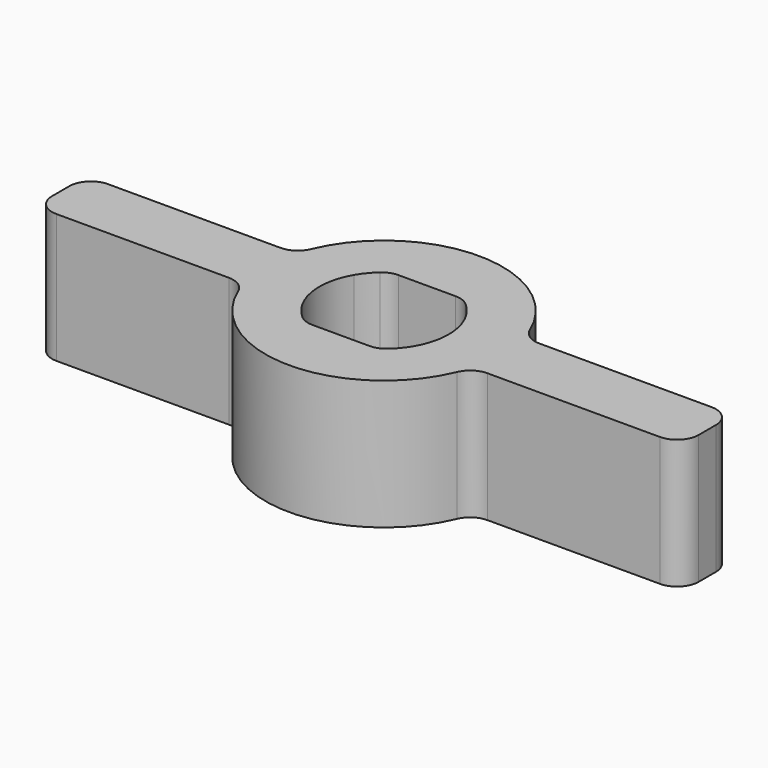
from build123d import *

# Parameters (mm, degrees)
F1_DEPTH = 6
F2_R     = 1
F3_R     = 1


with BuildPart() as f1:
    # F0 (on Top) → F1 (new body)
    with BuildSketch(Plane.XY):
        with BuildLine():
            ThreePointArc((-5.2915026221, -1.5), (0, -5.5), (5.2915026221, -1.5))
            Line((5.2915026221, -1.5), (2.5980762114, -1.5))
            ThreePointArc((2.5980762114, -1.5), (2.1861406616, -2.0544558909), (1.6583123952, -2.5))
            ThreePointArc((1.6583123952, -2.5), (0, -3), (-1.6583123952, -2.5))
            ThreePointArc((-1.6583123952, -2.5), (-2.1861406616, -2.0544558909), (-2.5980762114, -1.5))
            Line((-2.5980762114, -1.5), (-5.2915026221, -1.5))
        make_face()
        with BuildLine():
            ThreePointArc((-5.2915026221, -1.5), (-5.5, 0), (-5.2915026221, 1.5))
            Line((-5.2915026221, 1.5), (-15, 1.5))
            Line((-15, 1.5), (-15, -1.5))
            Line((-15, -1.5), (-5.2915026221, -1.5))
        make_face()
        with BuildLine():
            Line((-2.5980762114, 1.5), (-5.2915026221, 1.5))
            ThreePointArc((-5.2915026221, 1.5), (-5.5, 0), (-5.2915026221, -1.5))
            Line((-5.2915026221, -1.5), (-2.5980762114, -1.5))
            ThreePointArc((-2.5980762114, -1.5), (-3, 0), (-2.5980762114, 1.5))
        make_face()
        with BuildLine():
            ThreePointArc((5.2915026221, 1.5), (5.4476262914, 0.7572105316), (5.5, 0))
            ThreePointArc((5.5, 0), (5.4476262914, -0.7572105316), (5.2915026221, -1.5))
            Line((5.2915026221, -1.5), (15, -1.5))
            Line((15, -1.5), (15, 1.5))
            Line((15, 1.5), (5.2915026221, 1.5))
        make_face()
        with BuildLine():
            ThreePointArc((5.2915026221, -1.5), (5.4476262914, -0.7572105316), (5.5, 0))
            ThreePointArc((5.5, 0), (5.4476262914, 0.7572105316), (5.2915026221, 1.5))
            Line((5.2915026221, 1.5), (2.5980762114, 1.5))
            ThreePointArc((2.5980762114, 1.5), (2.8977774789, 0.7764571353), (3, 0))
            ThreePointArc((3, 0), (2.8977774789, -0.7764571353), (2.5980762114, -1.5))
            Line((2.5980762114, -1.5), (5.2915026221, -1.5))
        make_face()
        with BuildLine():
            Line((2.5980762114, 1.5), (5.2915026221, 1.5))
            ThreePointArc((5.2915026221, 1.5), (0, 5.5), (-5.2915026221, 1.5))
            Line((-5.2915026221, 1.5), (-2.5980762114, 1.5))
            ThreePointArc((-2.5980762114, 1.5), (-2.1861406616, 2.0544558909), (-1.6583123952, 2.5))
            ThreePointArc((-1.6583123952, 2.5), (0, 3), (1.6583123952, 2.5))
            ThreePointArc((1.6583123952, 2.5), (2.1861406616, 2.0544558909), (2.5980762114, 1.5))
        make_face()
        with BuildLine():
            Line((-1.6583123952, 2.5), (1.6583123952, 2.5))
            ThreePointArc((1.6583123952, 2.5), (0, 3), (-1.6583123952, 2.5))
        make_face()
        with BuildLine():
            ThreePointArc((-1.6583123952, -2.5), (0, -3), (1.6583123952, -2.5))
            Line((1.6583123952, -2.5), (-1.6583123952, -2.5))
        make_face()
    extrude(amount=F1_DEPTH)

    # F2
    f2_edges = [f1.edges().sort_by_distance(p)[0] for p in [
        (15, -1.5, 3),
        (-15, -1.5, 3),
        (15, 1.5, 3),
        (-15, 1.5, 3),
    ]]
    fillet(f2_edges, radius=F2_R)

    # F3
    f3_edges = [f1.edges().sort_by_distance(p)[0] for p in [
        (5.291503, -1.5, 3),
        (-5.291503, -1.5, 3),
        (-5.291503, 1.5, 3),
        (5.291503, 1.5, 3),
        (-1.658312, 2.5, 3),
        (1.658312, -2.5, 3),
        (1.658312, 2.5, 3),
        (-1.658312, -2.5, 3),
    ]]
    fillet(f3_edges, radius=F3_R)


solid = f1.part
